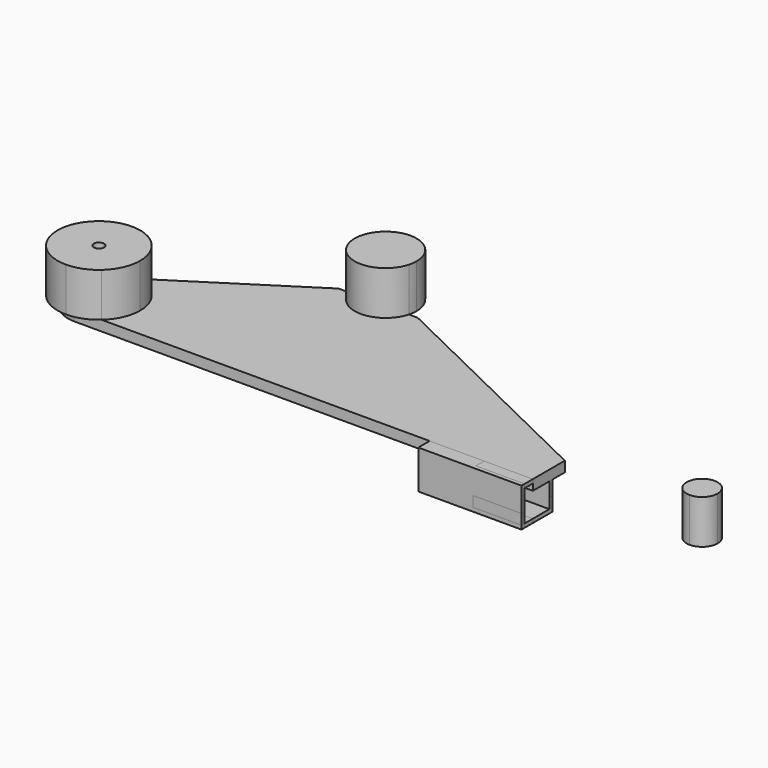
from build123d import *
from build123d import SkipClean  # not in build123d's __all__

# Parameters (mm, degrees)
F0_W            = 67.0499014769
F0_H            = 12.7
F0_H_2          = 4.7625
F0_W_2          = 59.9500985231
F0_H_3          = 25.7697334349
F1_DEPTH        = 47.625
F1_COPIES_COUNT = 2
F1_COPIES_ANGLE = 90
F2_W            = 38.1
F2_H            = 38.1
F3_DEPTH        = 127
F0_R            = 6.35
F0_W_3          = 339.3500985231
F4_DEPTH        = 12.7
F5_DEPTH        = 53.975


# Not quite as in the source:
# - a pattern or mirror of a feature is missing from the dataset's text; its kind, count and spacing are read off the source's solid
# - a feature names something its author has since deleted; it is built from what else it names


with BuildPart() as f1:
    # F0 (on Top) → F1 (new body)
    with BuildSketch(Plane.XY):
        with Locations((208.0981279893, -96.4646462023)):
            Rectangle(F0_W, F0_H)
        with Locations((208.0981279893, -105.1958962023)):
            Rectangle(F0_W, F0_H_2)
        with Locations((271.5981279893, -105.1958962023)):
            Rectangle(F0_W_2, F0_H_2)
        with Locations((208.0981279893, -77.2297794849)):
            Rectangle(F0_W, F0_H_3)
        Polygon((241.6230787277, -64.3449127674), (241.6230787277, -90.1146462023), (301.5731772508, -90.1146462023), (301.5731772508, -59.9521462023), (174.5731772508, -59.9521462023), (174.5731772508, -64.3449127674), align=None)
    extrude(amount=-F1_DEPTH)

    # F1_copies: F1 ×2 about axis
    f1_copies_axis = Axis((0, -83.764646, -23.8125), (1, 0, 0))


with BuildPart() as f1_1:
    add(f1.part, clean=False)
    with SkipClean():  # cleaning this boolean's faces spoils the solid; the shape is the same uncleaned
        for i in range(1, F1_COPIES_COUNT):
            add(f1.part.rotate(f1_copies_axis, i * F1_COPIES_ANGLE / (F1_COPIES_COUNT - 1)), clean=False)

    # F2 (on face) → F3 (cut, through all)
    with BuildSketch(Plane.YZ.offset(301.5731772508)):
        with Locations((-83.7646462023, -23.8125)):
            Rectangle(F2_W, F2_H)
    with SkipClean():  # cleaning this boolean's faces spoils the solid; the shape is the same uncleaned
        extrude(amount=-F3_DEPTH, mode=Mode.SUBTRACT)


with BuildPart() as f4:
    # F0 (on Top) → F4 (new body)
    with BuildSketch(Plane.XY):
        with BuildLine():
            Line((-91.8902158737, 102.9467433691), (-255.2069353227, -1.8036898565))
            ThreePointArc((-255.2069353227, -1.8036898565), (-224.3686917514, -18.9330173376), (-212.1205507423, -52.0146462023))
            ThreePointArc((-212.1205507423, -52.0146462023), (-216.6195090918, -72.9156878528), (-229.3195090918, -90.1146462023))
            Line((-229.3195090918, -90.1146462023), (-164.7769212723, -90.1146462023))
            Line((-164.7769212723, -90.1146462023), (-164.7769212723, -64.3449127674))
            Line((-164.7769212723, -64.3449127674), (174.5731772508, -64.3449127674))
            Line((174.5731772508, -64.3449127674), (174.5731772508, -59.9521462023))
            Line((174.5731772508, -59.9521462023), (301.5731772508, -59.9521462023))
            Line((301.5731772508, -59.9521462023), (301.5731772508, -40.9296154976))
            Line((301.5731772508, -40.9296154976), (5.4748591793, 102.9467433691))
            Line((5.4748591793, 102.9467433691), (-5.4159459459, 102.9467433691))
            ThreePointArc((-5.4159459459, 102.9467433691), (-42.1422114596, 74.9853537977), (-78.8684769732, 102.9467433691))
            Line((-78.8684769732, 102.9467433691), (-91.8902158737, 102.9467433691))
        make_face()
        with BuildLine():
            ThreePointArc((-212.1205507423, -52.0146462023), (-224.3686917514, -18.9330173376), (-255.2069353227, -1.8036898565))
            Line((-255.2069353227, -1.8036898565), (-283.4902114903, -19.9444254873))
            ThreePointArc((-283.4902114903, -19.9444254873), (-244.646170787, -18.5832681684), (-224.8205507423, -52.0146462023))
            ThreePointArc((-224.8205507423, -52.0146462023), (-235.9797823791, -78.9554145655), (-262.9205507423, -90.1146462023))
            Line((-262.9205507423, -90.1146462023), (-229.3195090918, -90.1146462023))
            ThreePointArc((-229.3195090918, -90.1146462023), (-216.6195090918, -72.9156878528), (-212.1205507423, -52.0146462023))
        make_face()
        with BuildLine():
            ThreePointArc((-224.8205507423, -52.0146462023), (-244.646170787, -18.5832681684), (-283.4902114903, -19.9444254873))
            ThreePointArc((-283.4902114903, -19.9444254873), (-299.4820428429, -62.7322623262), (-262.9205507423, -90.1146462023))
            ThreePointArc((-262.9205507423, -90.1146462023), (-235.9797823791, -78.9554145655), (-224.8205507423, -52.0146462023))
        make_face()
        with Locations((-262.9205507423, -52.0146462023)):
            Circle(F0_R, mode=Mode.SUBTRACT)
        with Locations((4.8981279893, -77.2297794849)):
            Rectangle(F0_W_3, F0_H_3)
        with BuildLine():
            Line((-5.4159459459, 102.9467433691), (-78.8684769732, 102.9467433691))
            ThreePointArc((-78.8684769732, 102.9467433691), (-42.1422114596, 74.9853537977), (-5.4159459459, 102.9467433691))
        make_face()
        with Locations((208.0981279893, -77.2297794849)):
            Rectangle(F0_W, F0_H_3)
        Polygon((241.6230787277, -64.3449127674), (241.6230787277, -90.1146462023), (301.5731772508, -90.1146462023), (301.5731772508, -59.9521462023), (174.5731772508, -59.9521462023), (174.5731772508, -64.3449127674), align=None)
    extrude(amount=-F4_DEPTH)


with BuildPart() as f5:
    # F0 (on Top) → F5 (new body)
    with BuildSketch(Plane.XY):
        with BuildLine():
            ThreePointArc((-28.0713410878, 148.4918589483), (-46.2820197032, 150.9597777234), (-63.5295651655, 144.616149878))
            ThreePointArc((-63.5295651655, 144.616149878), (-77.896694317, 126.2469249653), (-78.8684769732, 102.9467433691))
            Line((-78.8684769732, 102.9467433691), (-5.4159459459, 102.9467433691))
            ThreePointArc((-5.4159459459, 102.9467433691), (-4.3872070491, 107.9697265668), (-4.0422114596, 113.0853537977))
            ThreePointArc((-4.0422114596, 113.0853537977), (-10.6167442849, 134.4805616587), (-28.0713410878, 148.4918589483))
        make_face()
        with BuildLine():
            Line((-5.4159459459, 102.9467433691), (-78.8684769732, 102.9467433691))
            ThreePointArc((-78.8684769732, 102.9467433691), (-42.1422114596, 74.9853537977), (-5.4159459459, 102.9467433691))
        make_face()
    extrude(amount=F5_DEPTH)


with BuildPart() as f5b:
    # F0 (on Top) → F5, piece 2 (new body)
    with BuildSketch(Plane.XY):
        with BuildLine():
            ThreePointArc((-255.2069353227, -1.8036898565), (-274.0953662705, -2.4589855982), (-291.4370223503, -9.973584762))
            ThreePointArc((-291.4370223503, -9.973584762), (-311.4814708385, -66.9303104321), (-262.9205507423, -102.8146462023))
            ThreePointArc((-262.9205507423, -102.8146462023), (-244.9600385002, -99.5336950144), (-229.3195090918, -90.1146462023))
            Line((-229.3195090918, -90.1146462023), (-262.9205507423, -90.1146462023))
            ThreePointArc((-262.9205507423, -90.1146462023), (-299.4820428429, -62.7322623262), (-283.4902114903, -19.9444254873))
            Line((-283.4902114903, -19.9444254873), (-255.2069353227, -1.8036898565))
        make_face()
        with BuildLine():
            ThreePointArc((-224.8205507423, -52.0146462023), (-244.646170787, -18.5832681684), (-283.4902114903, -19.9444254873))
            ThreePointArc((-283.4902114903, -19.9444254873), (-299.4820428429, -62.7322623262), (-262.9205507423, -90.1146462023))
            ThreePointArc((-262.9205507423, -90.1146462023), (-235.9797823791, -78.9554145655), (-224.8205507423, -52.0146462023))
        make_face()
        with Locations((-262.9205507423, -52.0146462023)):
            Circle(F0_R, mode=Mode.SUBTRACT)
        with BuildLine():
            ThreePointArc((-212.1205507423, -52.0146462023), (-224.3686917514, -18.9330173376), (-255.2069353227, -1.8036898565))
            Line((-255.2069353227, -1.8036898565), (-283.4902114903, -19.9444254873))
            ThreePointArc((-283.4902114903, -19.9444254873), (-244.646170787, -18.5832681684), (-224.8205507423, -52.0146462023))
            ThreePointArc((-224.8205507423, -52.0146462023), (-235.9797823791, -78.9554145655), (-262.9205507423, -90.1146462023))
            Line((-262.9205507423, -90.1146462023), (-229.3195090918, -90.1146462023))
            ThreePointArc((-229.3195090918, -90.1146462023), (-216.6195090918, -72.9156878528), (-212.1205507423, -52.0146462023))
        make_face()
    extrude(amount=F5_DEPTH)


with BuildPart() as f5c:
    # F0 (on Top) → F5, piece 3 (new body)
    with BuildSketch(Plane.XY):
        with BuildLine():
            ThreePointArc((523.8231772508, -83.7646462023), (520.5359108382, -73.0670422718), (511.8086124367, -66.061393627))
            ThreePointArc((511.8086124367, -66.061393627), (486.0628931595, -80.1830586744), (504.7731772508, -102.8146462023))
            ThreePointArc((504.7731772508, -102.8146462023), (518.2435614324, -97.2350303839), (523.8231772508, -83.7646462023))
        make_face()
    extrude(amount=F5_DEPTH)


solid = Compound([f1_1.part, f4.part, f5.part, f5b.part, f5c.part])
